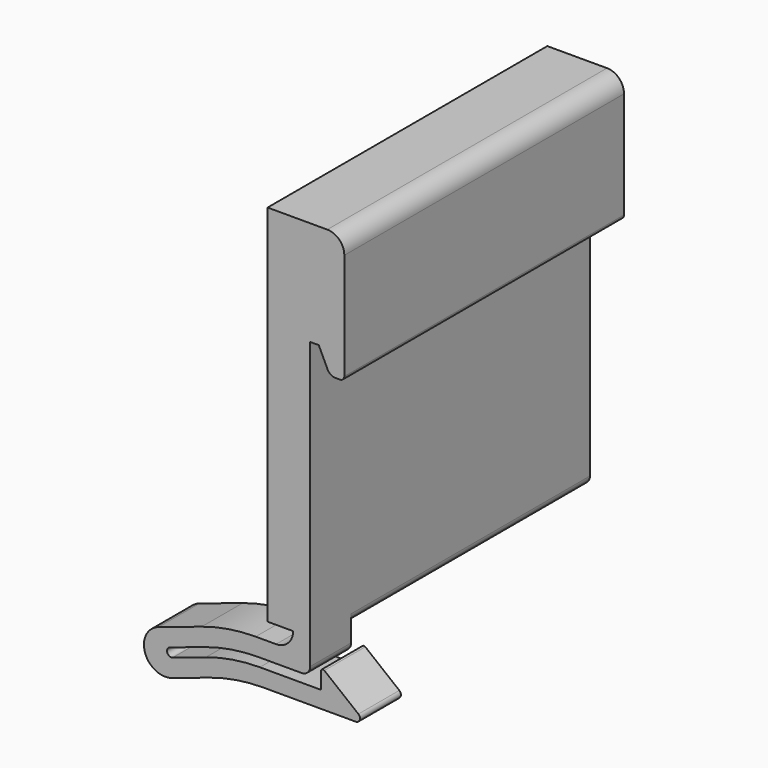
from build123d import *

# Parameters (mm, degrees)
F1_DEPTH = 6
F3_DEPTH = 35
F5_DEPTH = 3
F6_SIZE  = 2.99999


# Not quite as in the source:
# - a fillet or chamfer is up to 0.001 mm smaller than in the source, because OpenCascade refuses the exact size
# - ends of sketch curves that miss each other by under 0.0002 mm in the source are joined


with BuildPart() as f1:
    # F0 (on Front) → F1 (new body)
    with BuildSketch(Plane.XZ):
        with BuildLine():
            Line((14.498358, 10), (14.498358, 14))
            Line((14.498358, 14), (14.498358, 14.25))
            Line((14.498358, 14.25), (15.498358, 14.25))
            Line((15.498358, 14.25), (16.539344, 12.069217))
            ThreePointArc((16.539344, 12.069217), (16.908313, 11.654192), (17.4418, 11.5))
            Line((17.4418, 11.5), (17.998358, 11.5))
            ThreePointArc((17.998358, 11.5), (18.351911, 11.646447), (18.498358, 12))
            Line((18.498358, 12), (18.498358, 24.5))
            ThreePointArc((18.498358, 24.5), (17.912572, 25.914214), (16.498358, 26.5))
            Line((16.498358, 26.5), (14.498817, 26.5))
            Line((14.498817, 26.5), (12.498358, 26.5))
            Line((12.498358, 26.5), (12.498358, 24.5))
            Line((12.498358, 24.5), (12.498358, 22.5))
            Line((12.498358, 22.5), (12.498358, -16.25))
            ThreePointArc((12.498358, -16.25), (11.912572, -17.664214), (10.498358, -18.25))
            Line((10.498358, -18.25), (8.106805, -18.25))
            ThreePointArc((8.106805, -18.25), (4.90316, -18.508251), (1.78225, -19.276334))
            Line((1.78225, -19.276334), (-3.29057, -20.967274))
            ThreePointArc((-3.29057, -20.967274), (-4.871708, -24.129551), (-1.709431, -25.710691))
            Line((-1.709431, -25.710691), (2.709257, -24.237795))
            ThreePointArc((2.709257, -24.237795), (5.830167, -23.469711), (9.033812, -23.21146))
            Line((9.033812, -23.21146), (19.837293, -23.21146))
            ThreePointArc((19.837293, -23.21146), (20.309107, -22.876964), (20.149641, -22.321026))
            Line((20.149641, -22.321026), (16.154532, -19.124939))
            ThreePointArc((16.154532, -19.124939), (15.890061, -19.09483), (15.748358, -19.320156))
            Line((15.748358, -19.320156), (15.748358, -21.25))
            Line((15.748358, -21.25), (8.593639, -21.25))
            ThreePointArc((8.593639, -21.25), (5.389993, -21.508251), (2.269083, -22.276334))
            Line((2.269083, -22.276334), (-1.630813, -23.576299))
            ThreePointArc((-1.630813, -23.576299), (-2.263269, -23.260072), (-1.947041, -22.627616))
            Line((-1.947041, -22.627616), (2.106805, -21.276334))
            ThreePointArc((2.106805, -21.276334), (5.227716, -20.508251), (8.431361, -20.25))
            Line((8.431361, -20.25), (13.498358, -20.25))
            ThreePointArc((13.498358, -20.25), (14.205465, -19.957107), (14.498358, -19.25))
            Line((14.498358, -19.25), (14.498358, 10))
        make_face()
    extrude(amount=F1_DEPTH)

    # F2 (on face) → F3 (join)
    with BuildSketch(Plane(origin=(0, 0, 0), x_dir=(-1, 0, 0), z_dir=(0, 1, 0))):
        with BuildLine():
            ThreePointArc((-14.498358, -16.25), (-13.498358, -17.25), (-12.498358, -16.25))
            Line((-12.498358, -16.25), (-12.498358, 24.5))
            Line((-12.498358, 24.5), (-12.498358, 26.5))
            Line((-12.498358, 26.5), (-16.498358, 26.5))
            ThreePointArc((-16.498358, 26.5), (-17.912572, 25.914214), (-18.498358, 24.5))
            Line((-18.498358, 24.5), (-18.498358, 12))
            ThreePointArc((-18.498358, 12), (-18.351911, 11.646447), (-17.998358, 11.5))
            Line((-17.998358, 11.5), (-17.4418, 11.5))
            ThreePointArc((-17.4418, 11.5), (-16.908313, 11.654192), (-16.539344, 12.069217))
            Line((-16.539344, 12.069217), (-15.498358, 14.25))
            Line((-15.498358, 14.25), (-14.498358, 14.25))
            Line((-14.498358, 14.25), (-14.498358, -16.25))
        make_face()
    extrude(amount=F3_DEPTH)

    # F4 (on face) → F5 (join)
    with BuildSketch(Plane(origin=(12.498358, 0, 0), x_dir=(0, -1, 0), z_dir=(-1, 0, 0))):
        Polygon((-32, -16.25), (-32, 24.5), (4, 24.5), (4, -16.25), (6, -16.25), (6, 26.5), (-35, 26.5), (-35, -16.25), align=None)
    extrude(amount=F5_DEPTH)

    # F6 (size 3 in the source; OpenCascade refuses exactly that, so slightly less here)
    f6_edges = [f1.edges().sort_by_distance(p)[0] for p in [
        (9.498358, 32, 4.125),
    ]]
    chamfer(f6_edges, length=F6_SIZE)


solid = f1.part
